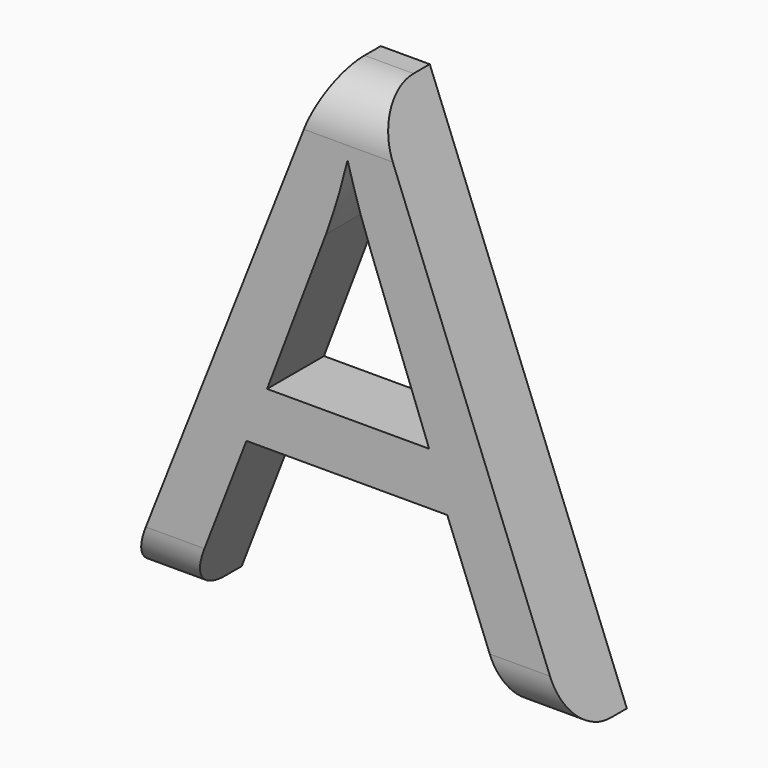
from build123d import *

# Parameters (mm, degrees)
F0_TEXT_SIZE = 17.5419069516
F1_DEPTH     = 1.778
F2_R         = 1.27


# Not quite as in the source:
# - Text() gives the source's letters only with a copy of the font that has no kerning and outlines rounded to 1/6400 em; it was checked with that copy


with BuildPart() as f1:
    # F0 (on Front) → F1 (new body)
    with BuildSketch(Plane.XZ):
        with Locations((-5.7814321481, -8.2539413124)):
            Text('A', F0_TEXT_SIZE, font='Open Sans', text_align=(TextAlign.LEFT, TextAlign.BOTTOM))
    extrude(amount=F1_DEPTH)

    # F2
    f2_edges = [f1.edges().sort_by_distance(p)[0] for p in [
        (-0.218729, -1.778, 4.321413),
        (-5.044124, -1.778, -8.253941),
        (4.565552, -1.778, -8.253941),
    ]]
    fillet(f2_edges, radius=F2_R)


solid = f1.part
